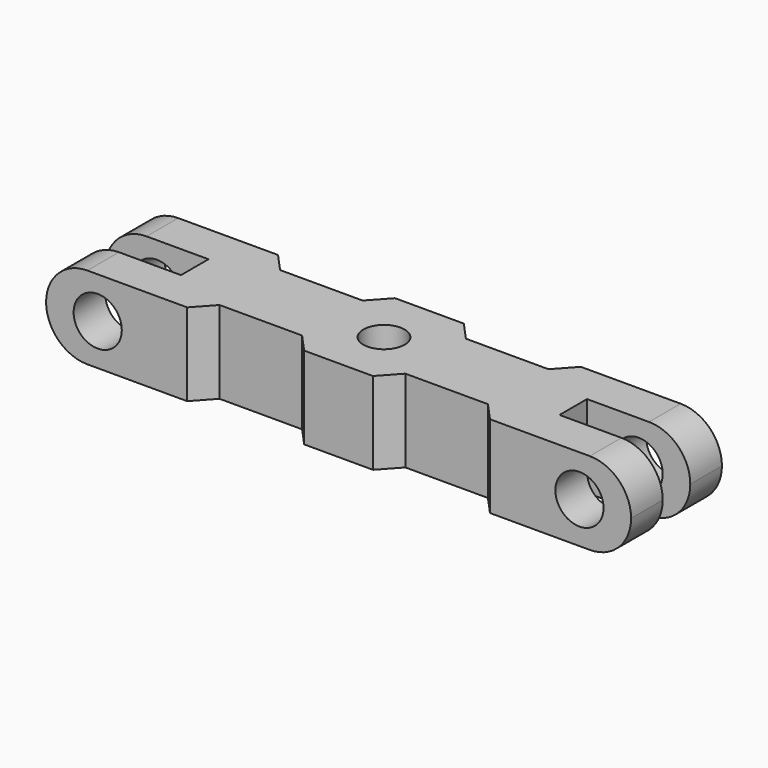
from build123d import *

# Parameters (mm, degrees)
F1_DEPTH = 12
F2_R     = 6
F3_DEPTH = 25
F4_R     = 7
F5_DEPTH = 50
F6_R     = 11.99999
F7_R     = 11.99999


# Not quite as in the source:
# - a fillet or chamfer is up to 0.001 mm smaller than in the source, because OpenCascade refuses the exact size


with BuildPart() as f1:
    # F0 (on Top) → F1 (new body, symmetric)
    with BuildSketch(Plane.XY):
        Polygon((10, 16.5), (0, 16.5), (-10, 16.5), (-15, 11), (-39, 11), (-44, 16.5), (-85, 16.5), (-85, 5), (-55, 5), (-55, 0), (-55, -5), (-85, -5), (-85, -16.5), (-44, -16.5), (-39, -11), (-15, -11), (-10, -16.5), (0, -16.5), (10, -16.5), (15, -11), (39, -11), (44, -16.5), (85, -16.5), (85, -5), (55, -5), (55, 0), (55, 5), (85, 5), (85, 16.5), (44, 16.5), (39, 11), (15, 11), align=None)
    extrude(amount=F1_DEPTH, both=True)

    # F2 (on Top) → F3 (cut, symmetric)
    with BuildSketch(Plane.XY):
        Circle(F2_R)
    extrude(amount=F3_DEPTH, both=True, mode=Mode.SUBTRACT)

    # F4 (on Front) → F5 (cut, symmetric)
    with BuildSketch(Plane.XZ):
        with Locations((70, 0)):
            Circle(F4_R)
        with Locations((-70, 0)):
            Circle(F4_R)
    extrude(amount=F5_DEPTH, both=True, mode=Mode.SUBTRACT)

    # F6 (radius 12 in the source; OpenCascade refuses exactly that, so slightly less here)
    f6_edges = [f1.edges().sort_by_distance(p)[0] for p in [
        (85, 10.75, 12),
        (85, -10.75, 12),
        (85, -10.75, -12),
        (85, 10.75, -12),
    ]]
    fillet(f6_edges, radius=F6_R)

    # F7 (radius 12 in the source; OpenCascade refuses exactly that, so slightly less here)
    f7_edges = [f1.edges().sort_by_distance(p)[0] for p in [
        (-85, -10.75, 12),
        (-85, 10.75, 12),
        (-85, 10.75, -12),
        (-85, -10.75, -12),
    ]]
    fillet(f7_edges, radius=F7_R)


solid = f1.part
